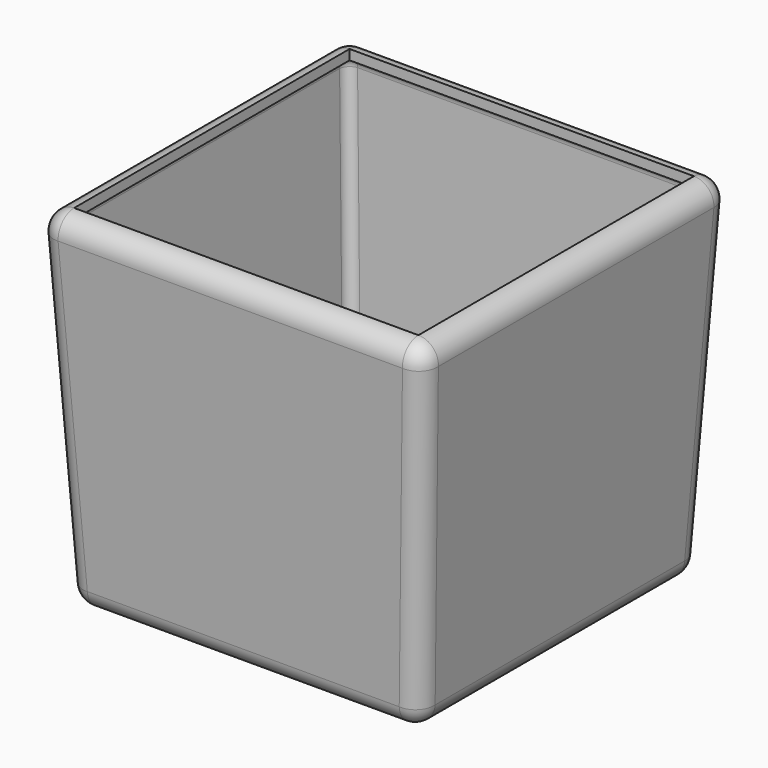
from build123d import *

# Parameters (mm, degrees)
F0_W                   = 88.9
F0_H                   = 88.9
F1_DEPTH               = 88.9
DRAFT_F1_DRAFTED_ANGLE = -3
F2_R                   = 5.08
F3_T                   = -2.54


# Not quite as in the source:
# - an extrude with a draft is written as a straight extrude whose walls are then drafted
# - a shell that OpenCascade refuses in one call is made with other operations: the cavity is built on its own and cut out


with BuildPart() as f1:
    # F0 (on Top) → F1 (new body)
    with BuildSketch(Plane.XY):
        with Locations((-3.1514364724, 1.4658318833)):
            Rectangle(F0_W, F0_H)
    extrude(amount=F1_DEPTH)

    # draft_F1_drafted
    draft_f1_drafted_walls = [f1.faces().sort_by_distance(p)[0] for p in [
        (-3.1514364724, 45.9158318833, 59.2666666667),
        (-47.6014364724, 1.4658318833, 59.2666666667),
        (-3.1514364724, -42.9841681167, 59.2666666667),
        (41.2985635276, 1.4658318833, 59.2666666667),
    ]]
    draft(draft_f1_drafted_walls, neutral_plane=Plane.XY, angle=DRAFT_F1_DRAFTED_ANGLE)

    # F2
    f2_edges = [f1.edges().sort_by_distance(p)[0] for p in [
        (43.628089, 48.245358, 44.45),
        (-49.930962, 48.245358, 44.45),
        (-3.151436, 45.915832, 0),
        (-3.151436, 50.574883, 88.9),
        (-49.930962, -45.313694, 44.45),
        (-47.601436, 1.465832, 0),
        (-52.260488, 1.465832, 88.9),
        (43.628089, -45.313694, 44.45),
        (-3.151436, -42.984168, 0),
        (-3.151436, -47.64322, 88.9),
        (41.298564, 1.465832, 0),
        (45.957615, 1.465832, 88.9),
    ]]
    fillet(f2_edges, radius=F2_R)

    # F3: a shell. OpenCascade refuses it in one call, so the cavity is built on its own and cut out:
    # the body offset inwards by the wall thickness, plus a prism from it out through each open face.
    f3_core = offset(f1.part, amount=F3_T, mode=Mode.PRIVATE)
    f3_exits = [f3_core.faces().sort_by_distance(p)[0] for p in [
        (-3.151436, 1.465832, 86.36),
    ]]
    add(f3_core, mode=Mode.SUBTRACT)
    extrude(f3_exits, amount=-F3_T, mode=Mode.SUBTRACT)


solid = f1.part
